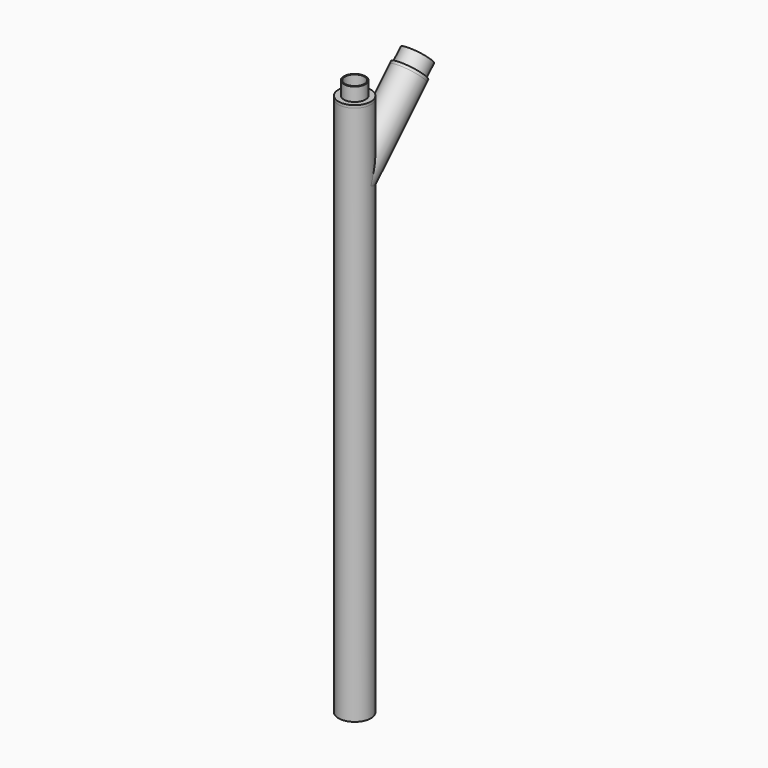
from build123d import *
from build123d import SkipClean  # not in build123d's __all__

# Parameters (mm, degrees)
F3_R      = 30
F3_R_2    = 27
F5_R      = 30
F5_R_2    = 27
F7_R      = 27
F8_DEPTH  = 1000.001
F9_R      = 27
F10_REACH = 885.9968684831
F11_R     = 30
F11_R_2   = 27
F12_DEPTH = 5
F13_R     = 20
F13_R_2   = 18
F14_DEPTH = 25
F15_R     = 18
F16_DEPTH = 25
F17_R     = 30
F17_R_2   = 27
F18_DEPTH = 5
F19_R     = 27
F19_R_2   = 25
F20_DEPTH = 25
F21_R     = 25
F22_DEPTH = 25


with BuildPart() as f4:
    # F4: sweep along a path in F0
    with BuildLine(Plane.YZ) as f4_path:
        Line((0, -487.5), (0, 380))
        Line((0, 380), (123.7436867076, 503.7436867076))
    # F3 (on plane+point) → F4 (sweep)
    with BuildSketch(Plane.XY.offset(-487.5)):
        Circle(F3_R)
        Circle(F3_R_2, mode=Mode.SUBTRACT)
    sweep(path=f4_path.line, transition=Transition.RIGHT)

    # F6: sweep along a path in F0
    with BuildLine(Plane.YZ) as f6_path:
        Line((0, 512.5), (0, 380))
    # F5 (on plane+point) → F6 (sweep)
    with BuildSketch(Plane.XY.offset(380)):
        Circle(F5_R)
        Circle(F5_R_2, mode=Mode.SUBTRACT)
    sweep(path=f6_path.line)

    # F7 (on face) → F8 (cut, through all)
    with BuildSketch(Plane.XY.offset(512.5)):
        Circle(F7_R)
    extrude(amount=-F8_DEPTH, mode=Mode.SUBTRACT)

    f10_end = f4.faces().sort_by_distance((-27, 0, 12.5))[0]
    # F9 (on face) → F10 (cut, up to a face of the model that its end follows)
    with BuildSketch(Plane(origin=(0, 313.7436867076, 313.7436867076), x_dir=(-1, 0, 0), z_dir=(0, 0.7071067812, 0.7071067812))):
        with Locations((0, 268.7005768509)):
            Circle(F9_R)
    f10_long = extrude(amount=-F10_REACH, mode=Mode.PRIVATE)
    add(split(f10_long, bisect_by=f10_end, keep=Keep.TOP, mode=Mode.PRIVATE), mode=Mode.SUBTRACT)

    # F11 (on face) → F12 (join)
    with BuildSketch(Plane.XY.offset(512.5)):
        Circle(F11_R)
        Circle(F11_R_2, mode=Mode.SUBTRACT)
        Circle(F11_R_2)
    with SkipClean():  # cleaning this boolean's faces spoils the solid; the shape is the same uncleaned
        extrude(amount=F12_DEPTH)

    # F13 (on face) → F14 (join)
    with BuildSketch(Plane.XY.offset(517.5)):
        Circle(F13_R)
        Circle(F13_R_2, mode=Mode.SUBTRACT)
    extrude(amount=F14_DEPTH)

    # F15 (on face) → F16 (cut)
    with BuildSketch(Plane.XY.offset(517.5)):
        Circle(F15_R)
    extrude(amount=-F16_DEPTH, mode=Mode.SUBTRACT)

    # F17 (on face) → F18 (join)
    with BuildSketch(Plane(origin=(0, 313.7436867076, 313.7436867076), x_dir=(-1, 0, 0), z_dir=(0, 0.7071067812, 0.7071067812))):
        with Locations((0, 268.7005768509)):
            Circle(F17_R)
        with Locations((0, 268.7005768509)):
            Circle(F17_R_2, mode=Mode.SUBTRACT)
        with Locations((0, 268.7005768509)):
            Circle(F17_R_2)
    extrude(amount=F18_DEPTH)

    # F19 (on face) → F20 (join)
    with BuildSketch(Plane(origin=(0, 317.2792206136, 317.2792206136), x_dir=(-1, 0, 0), z_dir=(0, 0.7071067812, 0.7071067812))):
        with Locations((0, 268.7005768509)):
            Circle(F19_R)
        with Locations((0, 268.7005768509)):
            Circle(F19_R_2, mode=Mode.SUBTRACT)
    extrude(amount=F20_DEPTH)

    # F21 (on face) → F22 (cut)
    with BuildSketch(Plane(origin=(0, 317.2792206136, 317.2792206136), x_dir=(-1, 0, 0), z_dir=(0, 0.7071067812, 0.7071067812))):
        with Locations((0, 268.7005768509)):
            Circle(F21_R)
    extrude(amount=-F22_DEPTH, mode=Mode.SUBTRACT)


solid = f4.part
